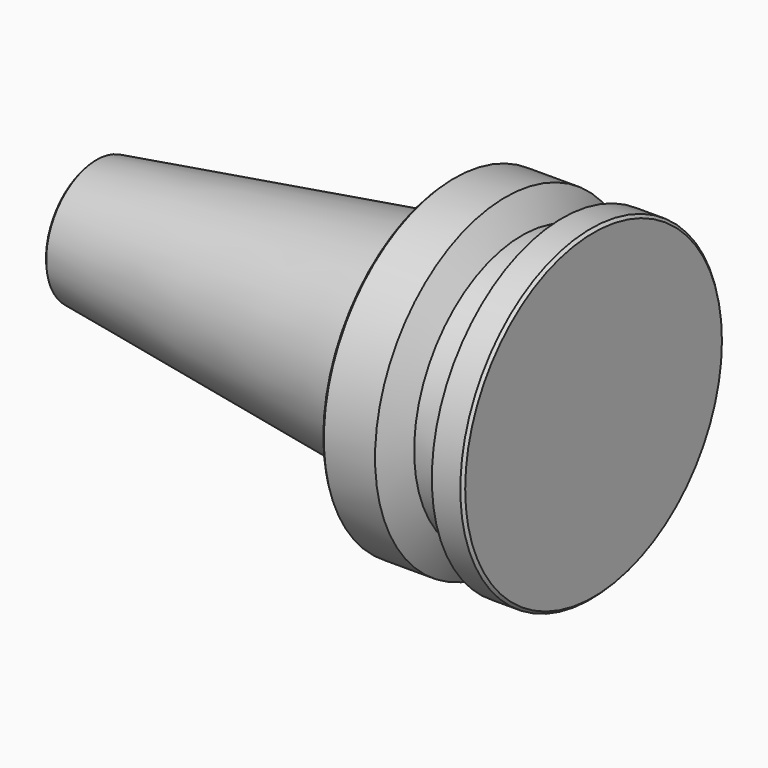
from build123d import *

# Parameters (mm, degrees)
F3_R = 0.254


# Not quite as in the source:
# - a fillet or chamfer that OpenCascade refuses, or shapes differently, is made with other operations: its cross-section is extruded or revolved along the edge and cut away or added


with BuildPart() as f1:
    # F0 (on Top) → F1 (revolve)
    with BuildSketch(Plane.XY):
        Polygon((-70.4, 0), (0, 0), (0, 23), (-4.4, 23), (-6.7094010768, 19), (-10.0905989232, 19), (-12.4, 23), (-20, 23), (-20, 14.875), (-22, 14.875), (-22, 15.875), (-70.4, 8.815), align=None)
    revolve(axis=Axis((-35.2, 0, 0), (1, 0, 0)))

    # F2: chamfer of 0.381 on 3 edges, made by hand

    # F2_s1 → F2_t2 (revolve, cut)
    with BuildSketch(Plane.XY):
        Polygon((0, 22.619), (-0.381, 23), (0, 23), align=None)
    revolve(axis=Axis((0, 0, 0), (1, 0, 0)), mode=Mode.SUBTRACT)

    # F2_s3 → F2_t4 (revolve, cut)
    with BuildSketch(Plane.XY):
        Polygon((-19.619, 23), (-20, 22.619), (-20, 23), align=None)
    revolve(axis=Axis((-20, 0, 0), (1, 0, 0)), mode=Mode.SUBTRACT)

    # F2_s5 → F2_t6 (revolve, cut)
    with BuildSketch(Plane.XY):
        Polygon((-70.4, 8.4855436088), (-70.0739936383, 8.8625538205), (-70.4, 8.815), align=None)
    revolve(axis=Axis((-70.4, 0, 0), (1, 0, 0)), mode=Mode.SUBTRACT)

    # F3
    f3_edges = [f1.edges().sort_by_distance(p)[0] for p in [
        (-22, -15.875, 0),
        (-22, -14.875, 0),
        (-20, -14.875, 0),
    ]]
    fillet(f3_edges, radius=F3_R)


solid = f1.part
